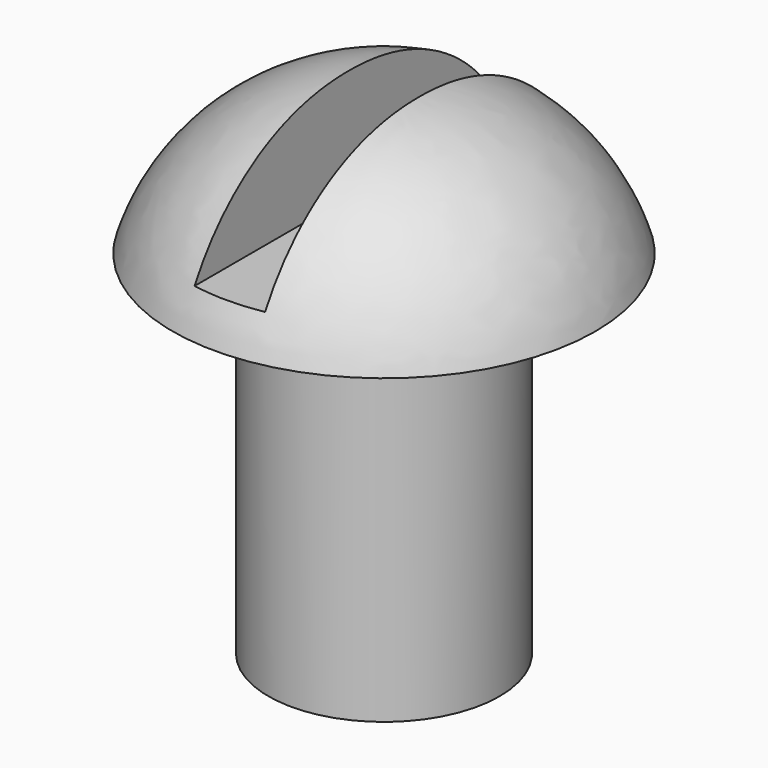
from build123d import *

# Parameters (mm, degrees)
F0_R     = 2.0828
F1_DEPTH = 6.35
F0_R_2   = 3.81
F2_DEPTH = 2.7178
F4_W     = 1.27
F4_H     = 4.064
F5_DEPTH = 3.81


# Not quite as in the source:
# - a fillet or chamfer that OpenCascade refuses, or shapes differently, is made with other operations: its cross-section is extruded or revolved along the edge and cut away or added


with BuildPart() as f1:
    # F0 (on Top) → F1 (new body)
    with BuildSketch(Plane.XY):
        Circle(F0_R)
    extrude(amount=-F1_DEPTH)

    # F0 (on Top) → F2 (join)
    with BuildSketch(Plane.XY):
        Circle(F0_R_2)
        Circle(F0_R, mode=Mode.SUBTRACT)
        Circle(F0_R)
    extrude(amount=F2_DEPTH)

    # F3: fillet of radius 3.81 on 1 edges, made by hand

    # F3_s1 → F3_t2 (revolve, cut)
    with BuildSketch(Plane.XZ):
        with BuildLine():
            ThreePointArc((3.81, 0), (2.43529628, 1.9637271915), (0.1599042259, 2.7178))
            Line((0.1599042259, 2.7178), (3.81, 2.7178))
            Line((3.81, 2.7178), (3.81, 0))
        make_face()
    revolve(axis=Axis((0, 0, 2.7178), (0, 0, 1)), mode=Mode.SUBTRACT)

    # F4 (on Front) → F5 (cut, symmetric)
    with BuildSketch(Plane.XZ):
        with Locations((0, 2.7178)):
            Rectangle(F4_W, F4_H)
    extrude(amount=F5_DEPTH, both=True, mode=Mode.SUBTRACT)


solid = f1.part
